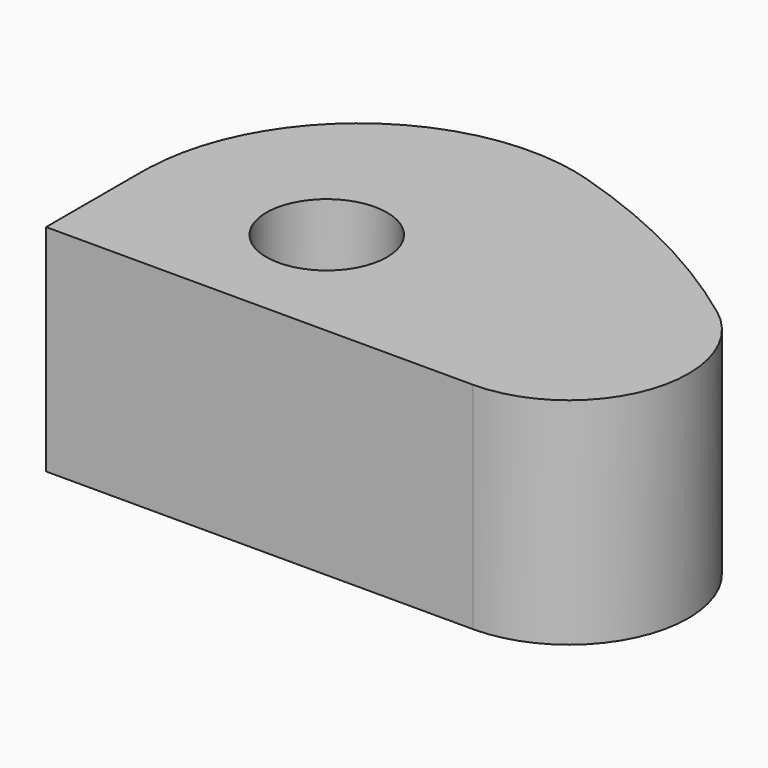
from build123d import *

# Parameters (mm, degrees)
F0_R        = 5.05
F1_DEPTH    = 18
F2_R        = 10
F3_T1_DEPTH = 139.38722981
F4_R        = 9.99999
F5_T1_DEPTH = 121.084516093
F6_R        = 18


# Not quite as in the source:
# - a fillet or chamfer that OpenCascade refuses, or shapes differently, is made with other operations: its cross-section is extruded or revolved along the edge and cut away or added
# - a fillet or chamfer is up to 0.001 mm smaller than in the source, because OpenCascade refuses the exact size


with BuildPart() as f1:
    # F0 (on Top) → F1 (new body)
    with BuildSketch(Plane.XY):
        Polygon((-17.3258748727, 30), (-17.3258748727, 0), (42.6741251273, 0), (12.6741251273, 30), align=None)
        with Locations((-2.3258748727, 10.59)):
            Circle(F0_R, mode=Mode.SUBTRACT)
    extrude(amount=F1_DEPTH)

    # F2
    f2_edges = [f1.edges().sort_by_distance(p)[0] for p in [
        (42.674125, 0, 9),
    ]]
    fillet(f2_edges, radius=F2_R)

    # F3: fillet of radius 60 on 1 edges, made by hand

    # F3_s2 → F3_t1 (cut)
    with BuildSketch(Plane.XY.offset(-60.693614905)):
        with BuildLine():
            ThreePointArc((25.6030573154, 17.0710678119), (8.0910429692, 26.6756740971), (-11.6033208347, 30))
            Line((-11.6033208347, 30), (-11.6033208347, 31.2))
            Line((-11.6033208347, 31.2), (12.6741251273, 31.2))
            Line((12.6741251273, 31.2), (13.5226532647, 30.8485281374))
            ThreePointArc((13.5226532647, 30.8485281374), (19.9871193587, 24.3840620434), (26.3471848784, 18.0124891681))
            Line((26.3471848784, 18.0124891681), (25.6030573154, 17.0710678119))
        make_face()
    extrude(amount=F3_T1_DEPTH, mode=Mode.SUBTRACT)

    # F4 (radius 10 in the source; OpenCascade refuses exactly that, so slightly less here)
    f4_edges = [f1.edges().sort_by_distance(p)[0] for p in [
        (25.603057, 17.071068, 9),
    ]]
    fillet(f4_edges, radius=F4_R)

    # F5: fillet of radius 40 on 1 edges, made by hand

    # F5_s2 → F5_t1 (cut)
    with BuildSketch(Plane.XY.offset(-51.5422580465)):
        with BuildLine():
            ThreePointArc((-17.3258748727, 9.3830967814), (-15.8686941682, 20.0812779708), (-11.6033208347, 30))
            Line((-11.6033208347, 30), (-17.3258748727, 30))
            Line((-17.3258748727, 30), (-17.3258748727, 9.3830967814))
        make_face()
    extrude(amount=F5_T1_DEPTH, mode=Mode.SUBTRACT)

    # F6
    f6_edges = [f1.edges().sort_by_distance(p)[0] for p in [
        (-11.603321, 30, 9),
    ]]
    fillet(f6_edges, radius=F6_R)


solid = f1.part
